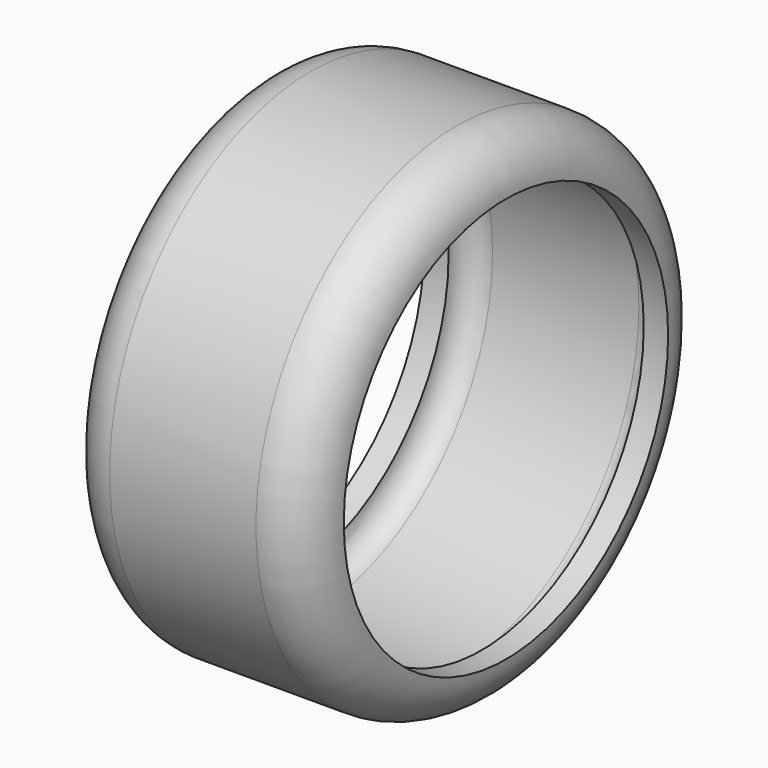
from build123d import *

# Parameters (mm, degrees)
F0_R     = 26.1896529573
F1_DEPTH = 25.4
F2_R     = 5.08
F3_T     = -2.54


# Not quite as in the source:
# - a shell that OpenCascade refuses in one call is made with other operations: the cavity is built on its own and cut out


with BuildPart() as f1:
    # F0 (on Right) → F1 (new body)
    with BuildSketch(Plane.YZ):
        with Locations((-9.9267605692, 26.3711642474)):
            Circle(F0_R)
    extrude(amount=F1_DEPTH)

    # F2
    f2_edges = [f1.edges().sort_by_distance(p)[0] for p in [
        (25.4, -36.116414, 26.371164),
        (0, -36.116414, 26.371164),
        (12.7, 16.262892, 26.371164),
    ]]
    fillet(f2_edges, radius=F2_R)

    # F3: a shell. OpenCascade refuses it in one call, so the cavity is built on its own and cut out:
    # the body offset inwards by the wall thickness, plus a prism from it out through each open face.
    f3_core = offset(f1.part, amount=F3_T, mode=Mode.PRIVATE)
    f3_exits = [f3_core.faces().sort_by_distance(p)[0] for p in [
        (22.86, -9.926761, 26.371164),
        (2.54, -9.926761, 26.371164),
    ]]
    add(f3_core, mode=Mode.SUBTRACT)
    extrude(f3_exits, amount=-F3_T, mode=Mode.SUBTRACT)


solid = f1.part
